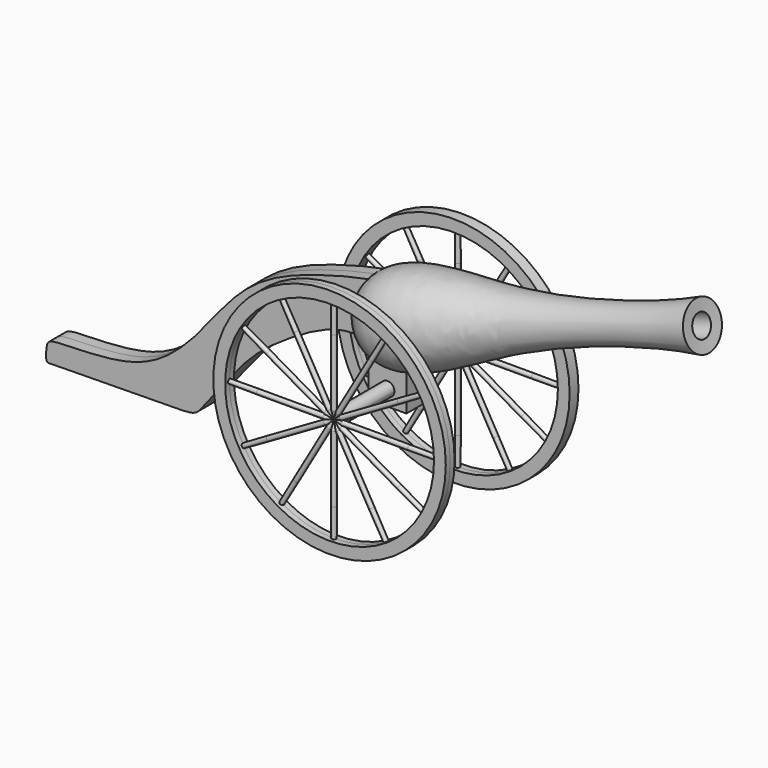
from build123d import *

# Parameters (mm, degrees)
F2_W          = 174.1611883044
F2_H          = 96.2469726801
F3_DEPTH      = 299.72
F5_DEPTH      = 50.8
F5_DEPTH_BACK = 50.8
F7_DEPTH      = 355.6
F7_DEPTH_BACK = 355.6
F8_R          = 533.9093393736
F8_R_2        = 479.7664821329
F9_DEPTH      = 25.4
F9_DEPTH_BACK = 25.4
F12_COUNT     = 12


with BuildPart() as f1:
    # F0 (on Front) → F1 (revolve)
    with BuildSketch(Plane.XZ):
        with BuildLine():
            add(Edge.make_bspline(
                [(0, 0), (-25.50103474, 77.3661173144), (42.3630253812, 294.8010438764), (652.0761470543, 297.0371774632), (1189.0276313793, 437.2149051763), (1422.8546228763, 523.6061963171), (1516.9641971588, 566.6810274124)],
                knots=[0, 0, 0, 0, 0.1844356068, 0.4770909986, 0.7740481254, 1, 1, 1, 1], degree=3))
            Line((0, 0), (109.6523288958, 33.0051883212))
            add(Edge.make_bspline(
                [(548.6290850142, 218.1878955915), (506.3855943503, 208.8531126129), (415.7069187368, 188.8153329612), (252.2689061049, 216.0363104908), (68.0569758496, 159.3694539532), (96.6479694606, 72.5116766593), (109.6523288958, 33.0051883212)],
                knots=[0, 0, 0, 0, 0.2416708383, 0.5187637482, 0.7811139663, 1, 1, 1, 1], degree=3))
            Line((548.6290850142, 218.1878955915), (1528.9520563061, 513.2636555768))
            Line((1528.9520563061, 513.2636555768), (1516.9641971588, 566.6810274124))
        make_face()
    revolve(axis=Axis((54.8261644479, 0, 16.5025941606), (0.9575627252, 0, 0.2882249597)))

    # F2 (on Top) → F3 (join)
    with BuildSketch(Plane.XY):
        with Locations((138.9069408178, 0)):
            Rectangle(F2_W, F2_H)
    extrude(amount=-F3_DEPTH)

    # F4 (on Front) → F5 (join, two sides)
    with BuildSketch(Plane.XZ) as f5_sk:
        with BuildLine():
            add(Edge.make_bspline(
                [(98.8123938441, 191.9083893299), (88.9082757739, 201.3209173099), (-391.313434187, 99.1788598763), (-632.7674605201, -150.5583359951), (-927.6049619509, -563.041976897), (-1404.9188815055, -515.757230428), (-1425.5571354063, -557.3145811799), (-1429.7525917928, -629.1185921879), (-1394.650601474, -627.328760558), (-832.0731036085, -619.5158426609), (-830.4726459204, -619.8336063892), (-746.1775841659, -620.4955124915), (-704.6804410819, -577.7411166643), (-517.0312716334, -321.5223490711), (-360.572346845, -194.4520087919), (-77.4211971302, -25.5089768496), (66.4198516221, -65.9834857173), (60.7259063147, -31.3418637323), (14.3532427818, 27.0502464301), (37.5504052453, 160.7860578394), (102.2696100116, 188.6227718041), (98.8123938441, 191.9083893299)],
                knots=[0, 0, 0, 0, 0.086896341, 0.1716992731, 0.2639127657, 0.3489768844, 0.3729076209, 0.4051418339, 0.428950155, 0.5278522472, 0.5439662628, 0.5788207851, 0.611845586, 0.684483741, 0.7486084683, 0.8241381899, 0.8687581692, 0.8857438125, 0.9213178606, 0.96966722, 1, 1, 1, 1], degree=3))
        make_face()
    extrude(amount=F5_DEPTH)
    extrude(f5_sk.sketch, amount=-F5_DEPTH_BACK)

    # F6 (on Front) → F7 (join, two sides)
    with BuildSketch(Plane.XZ) as f7_sk:
        with BuildLine():
            ThreePointArc((139.4005864859, -259.5243079525), (161.8512267885, -250.2249482552), (171.1505864859, -227.7743079525))
            ThreePointArc((171.1505864859, -227.7743079525), (116.9499461832, -205.3236676498), (139.4005864859, -259.5243079525))
        make_face()
    extrude(amount=F7_DEPTH)
    extrude(f7_sk.sketch, amount=-F7_DEPTH_BACK)


with BuildPart() as f9:
    # F8 (on face) → F9 (new body, two sides)
    with BuildSketch(Plane.XZ.offset(355.6)) as f9_sk:
        with Locations((139.4005864859, -227.7743079525)):
            Circle(F8_R)
        with Locations((139.4005864859, -227.7743079525)):
            Circle(F8_R_2, mode=Mode.SUBTRACT)
    extrude(amount=-F9_DEPTH)
    extrude(f9_sk.sketch, amount=F9_DEPTH_BACK)


with BuildPart() as f11:
    # F10 (on face) → F11 (revolve)
    with BuildSketch(Plane.XZ.offset(355.6)):
        Polygon((150.2021700144, -269.1336608153), (139.4005864859, -227.7743079525), (139.4005864859, -731.6109538078), (149.148657918, -731.6109538078), (150.2021700144, -575.1153230667), align=None)
    revolve(axis=Axis((139.4005864859, -355.6, -479.6926308802), (0, 0, -1)))


with BuildPart() as f12_1:
    # F12: instance of F11
    add(f11.part.rotate(Axis((139.4005864859, -355.6, -227.7743079525), (0, 1, 0)), 1 * 360 / F12_COUNT))


with BuildPart() as f12_2:
    # F12: instance of F11
    add(f11.part.rotate(Axis((139.4005864859, -355.6, -227.7743079525), (0, 1, 0)), 2 * 360 / F12_COUNT))


with BuildPart() as f12_3:
    # F12: instance of F11
    add(f11.part.rotate(Axis((139.4005864859, -355.6, -227.7743079525), (0, 1, 0)), 3 * 360 / F12_COUNT))


with BuildPart() as f12_4:
    # F12: instance of F11
    add(f11.part.rotate(Axis((139.4005864859, -355.6, -227.7743079525), (0, 1, 0)), 4 * 360 / F12_COUNT))


with BuildPart() as f12_5:
    # F12: instance of F11
    add(f11.part.rotate(Axis((139.4005864859, -355.6, -227.7743079525), (0, 1, 0)), 5 * 360 / F12_COUNT))


with BuildPart() as f12_6:
    # F12: instance of F11
    add(f11.part.rotate(Axis((139.4005864859, -355.6, -227.7743079525), (0, 1, 0)), 6 * 360 / F12_COUNT))


with BuildPart() as f12_7:
    # F12: instance of F11
    add(f11.part.rotate(Axis((139.4005864859, -355.6, -227.7743079525), (0, 1, 0)), 7 * 360 / F12_COUNT))


with BuildPart() as f12_8:
    # F12: instance of F11
    add(f11.part.rotate(Axis((139.4005864859, -355.6, -227.7743079525), (0, 1, 0)), 8 * 360 / F12_COUNT))


with BuildPart() as f12_9:
    # F12: instance of F11
    add(f11.part.rotate(Axis((139.4005864859, -355.6, -227.7743079525), (0, 1, 0)), 9 * 360 / F12_COUNT))


with BuildPart() as f12_10:
    # F12: instance of F11
    add(f11.part.rotate(Axis((139.4005864859, -355.6, -227.7743079525), (0, 1, 0)), 10 * 360 / F12_COUNT))


with BuildPart() as f12_11:
    # F12: instance of F11
    add(f11.part.rotate(Axis((139.4005864859, -355.6, -227.7743079525), (0, 1, 0)), 11 * 360 / F12_COUNT))


with BuildPart() as f13_1:
    # F13: instance of F9
    add(f9.part.mirror(Plane.XZ))


with BuildPart() as f13_2:
    # F13: instance of F12_4
    add(f12_4.part.mirror(Plane.XZ))


with BuildPart() as f13_3:
    # F13: instance of F12_3
    add(f12_3.part.mirror(Plane.XZ))


with BuildPart() as f13_4:
    # F13: instance of F12_2
    add(f12_2.part.mirror(Plane.XZ))


with BuildPart() as f13_5:
    # F13: instance of F12_1
    add(f12_1.part.mirror(Plane.XZ))


with BuildPart() as f13_6:
    # F13: instance of F11
    add(f11.part.mirror(Plane.XZ))


with BuildPart() as f13_7:
    # F13: instance of F12_11
    add(f12_11.part.mirror(Plane.XZ))


with BuildPart() as f13_8:
    # F13: instance of F12_10
    add(f12_10.part.mirror(Plane.XZ))


with BuildPart() as f13_9:
    # F13: instance of F12_9
    add(f12_9.part.mirror(Plane.XZ))


with BuildPart() as f13_10:
    # F13: instance of F12_8
    add(f12_8.part.mirror(Plane.XZ))


with BuildPart() as f13_11:
    # F13: instance of F12_7
    add(f12_7.part.mirror(Plane.XZ))


with BuildPart() as f13_12:
    # F13: instance of F12_6
    add(f12_6.part.mirror(Plane.XZ))


with BuildPart() as f13_13:
    # F13: instance of F12_5
    add(f12_5.part.mirror(Plane.XZ))


solid = Compound([f1.part, f9.part, f11.part, f12_1.part, f12_2.part, f12_3.part, f12_4.part, f12_5.part, f12_6.part, f12_7.part, f12_8.part, f12_9.part, f12_10.part, f12_11.part, f13_1.part, f13_2.part, f13_3.part, f13_4.part, f13_5.part, f13_6.part, f13_7.part, f13_8.part, f13_9.part, f13_10.part, f13_11.part, f13_12.part, f13_13.part])
